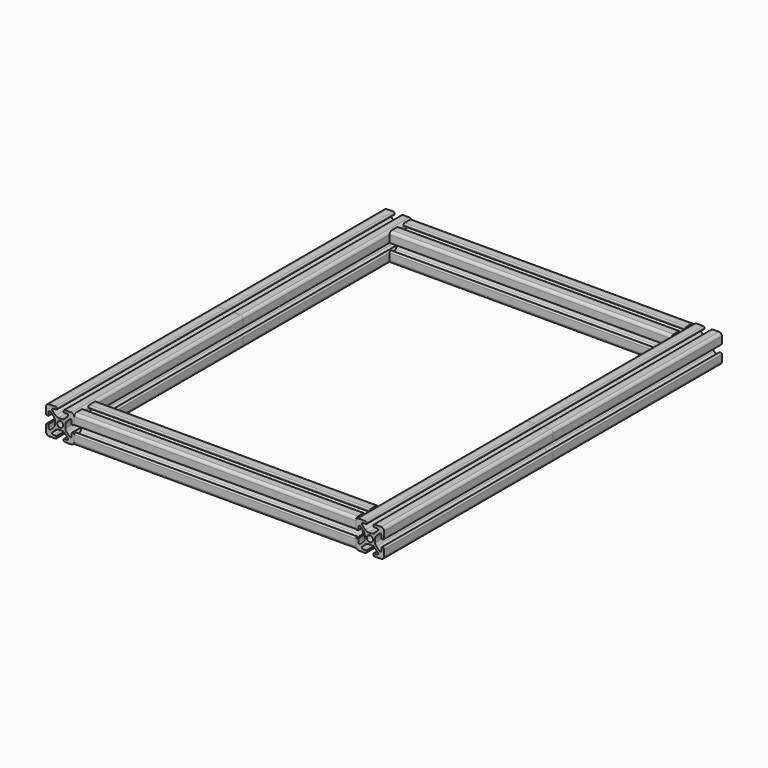
from build123d import *

# Parameters (mm, degrees)
F1_DEPTH = 150
F3_DEPTH = 100


# Not quite as in the source:
# - ends of sketch curves that miss each other by under 0.0002 mm in the source are joined


with BuildPart() as f1:
    # F0 (on Front) → F1 (new body, symmetric)
    with BuildSketch(Plane.XZ):
        with BuildLine():
            ThreePointArc((-112.15, 0), (-111.5202795796, 1.5202795796), (-110, 2.15))
            Line((-110, 2.15), (-110, 3.65))
            Line((-110, 3.65), (-111.134567, 3.65))
            ThreePointArc((-111.134567, 3.65), (-112.2826172971, 3.8783614025), (-113.2558873436, 4.5286796564))
            Line((-113.2558873436, 4.5286796564), (-115.506192, 6.778984))
            ThreePointArc((-115.506192, 6.778984), (-115.6866364094, 7.6861382813), (-114.917588, 8.2))
            Line((-114.917588, 8.2), (-112.8, 8.200001))
            ThreePointArc((-112.8, 8.200001), (-112.5878679656, 8.2878679656), (-112.5, 8.5))
            Line((-112.5, 8.5), (-112.5, 9.200001))
            ThreePointArc((-112.5, 9.200001), (-112.7343145751, 9.7656854249), (-113.3, 10))
            Line((-113.3, 10), (-118, 10))
            ThreePointArc((-118, 10), (-119.4142135624, 9.4142135624), (-120, 8))
            Line((-120, 8), (-120, 3.3))
            ThreePointArc((-120, 3.3), (-119.7656854249, 2.7343145751), (-119.2, 2.5))
            Line((-119.2, 2.5), (-118.5, 2.5))
            ThreePointArc((-118.5, 2.5), (-118.2878679656, 2.5878679656), (-118.2, 2.8))
            Line((-118.2, 2.8), (-118.2, 4.917588))
            ThreePointArc((-118.2, 4.917588), (-117.6861382813, 5.6866364094), (-116.7789838301, 5.5061921699))
            Line((-116.7789838301, 5.5061921699), (-114.52868, 3.255887))
            ThreePointArc((-114.52868, 3.255887), (-113.8783614025, 2.2826172971), (-113.65, 1.134567))
            Line((-113.65, 1.134567), (-113.65, 0))
            Line((-113.65, 0), (-112.15, 0))
        make_face()
        with BuildLine():
            Line((-107.85, 0), (-106.35, 0))
            Line((-106.35, 0), (-106.35, 1.134567))
            ThreePointArc((-106.35, 1.134567), (-106.1216385975, 2.2826172971), (-105.4713203436, 3.2558873436))
            Line((-105.4713203436, 3.2558873436), (-103.221016, 5.506192))
            ThreePointArc((-103.221016, 5.506192), (-102.3138617187, 5.6866364094), (-101.8, 4.917588))
            Line((-101.8, 4.917588), (-101.799999, 2.8))
            ThreePointArc((-101.799999, 2.8), (-101.7121320344, 2.5878679656), (-101.5, 2.5))
            Line((-101.5, 2.5), (-100.799999, 2.5))
            ThreePointArc((-100.799999, 2.5), (-100.2343145751, 2.7343145751), (-100, 3.3))
            Line((-100, 3.3), (-100, 8))
            ThreePointArc((-100, 8), (-100.5857864376, 9.4142135624), (-102, 10))
            Line((-102, 10), (-106.7, 10))
            ThreePointArc((-106.7, 10), (-107.2656854249, 9.7656854249), (-107.5, 9.2))
            Line((-107.5, 9.2), (-107.5, 8.5))
            ThreePointArc((-107.5, 8.5), (-107.4121320344, 8.2878679656), (-107.2, 8.2))
            Line((-107.2, 8.2), (-105.082412, 8.200001))
            ThreePointArc((-105.082412, 8.200001), (-104.3133635906, 7.6861382813), (-104.4938078301, 6.7789838301))
            Line((-104.4938078301, 6.7789838301), (-106.744113, 4.52868))
            ThreePointArc((-106.744113, 4.52868), (-107.7173827029, 3.8783614025), (-108.865433, 3.65))
            Line((-108.865433, 3.65), (-110, 3.65))
            Line((-110, 3.65), (-110, 2.15))
            ThreePointArc((-110, 2.15), (-108.4797204204, 1.5202795796), (-107.85, 0))
        make_face()
        with BuildLine():
            Line((-110, -3.65), (-110, -2.15))
            ThreePointArc((-110, -2.15), (-111.5202795796, -1.5202795796), (-112.15, 0))
            Line((-112.15, 0), (-113.65, 0))
            Line((-113.65, 0), (-113.65, -1.134567))
            ThreePointArc((-113.65, -1.134567), (-113.8783614025, -2.2826172971), (-114.5286796564, -3.2558873436))
            Line((-114.5286796564, -3.2558873436), (-116.778985, -5.506192))
            ThreePointArc((-116.778985, -5.506192), (-117.6861382813, -5.6866364094), (-118.2, -4.917588))
            Line((-118.2, -4.917588), (-118.2, -2.8))
            ThreePointArc((-118.2, -2.8), (-118.2878679656, -2.5878679656), (-118.5, -2.5))
            Line((-118.5, -2.5), (-119.2, -2.5))
            ThreePointArc((-119.2, -2.5), (-119.7656854249, -2.7343145751), (-120, -3.3))
            Line((-120, -3.3), (-120, -8))
            ThreePointArc((-120, -8), (-119.4142135624, -9.4142135624), (-118, -10))
            Line((-118, -10), (-113.3, -10))
            ThreePointArc((-113.3, -10), (-112.7343145751, -9.7656854249), (-112.5, -9.2))
            Line((-112.5, -9.2), (-112.5, -8.5))
            ThreePointArc((-112.5, -8.5), (-112.5878679656, -8.2878679656), (-112.8, -8.2))
            Line((-112.8, -8.2), (-114.917588, -8.2))
            ThreePointArc((-114.917588, -8.2), (-115.6866364094, -7.6861382813), (-115.5061921699, -6.7789838301))
            Line((-115.5061921699, -6.7789838301), (-113.255888, -4.52868))
            ThreePointArc((-113.255888, -4.52868), (-112.2826172971, -3.8783614025), (-111.134567, -3.65))
            Line((-111.134567, -3.65), (-110, -3.65))
        make_face()
        with BuildLine():
            ThreePointArc((-101.8, -4.917588), (-102.3138617187, -5.6866364094), (-103.2210161699, -5.5061921699))
            Line((-103.2210161699, -5.5061921699), (-105.47132, -3.255888))
            ThreePointArc((-105.47132, -3.255888), (-106.1216385975, -2.2826172971), (-106.35, -1.134567))
            Line((-106.35, -1.134567), (-106.35, 0))
            Line((-106.35, 0), (-107.85, 0))
            ThreePointArc((-107.85, 0), (-108.4797204204, -1.5202795796), (-110, -2.15))
            Line((-110, -2.15), (-110, -3.65))
            Line((-110, -3.65), (-108.865433, -3.65))
            ThreePointArc((-108.865433, -3.65), (-107.7173827029, -3.8783614025), (-106.7441126564, -4.5286796564))
            Line((-106.7441126564, -4.5286796564), (-104.493808, -6.778985))
            ThreePointArc((-104.493808, -6.778985), (-104.3133635906, -7.6861382813), (-105.082412, -8.2))
            Line((-105.082412, -8.2), (-107.2, -8.2))
            ThreePointArc((-107.2, -8.2), (-107.4121320344, -8.2878679656), (-107.5, -8.5))
            Line((-107.5, -8.5), (-107.5, -9.2))
            ThreePointArc((-107.5, -9.2), (-107.2656854249, -9.7656854249), (-106.7, -10))
            Line((-106.7, -10), (-102, -10))
            ThreePointArc((-102, -10), (-100.5857864376, -9.4142135624), (-100, -8))
            Line((-100, -8), (-100, -3.3))
            ThreePointArc((-100, -3.3), (-100.2343145751, -2.7343145751), (-100.8, -2.5))
            Line((-100.8, -2.5), (-101.5, -2.5))
            ThreePointArc((-101.5, -2.5), (-101.7121320344, -2.5878679656), (-101.8, -2.8))
            Line((-101.8, -2.8), (-101.8, -4.917588))
        make_face()
    extrude(amount=F1_DEPTH, both=True)


with BuildPart() as f1b:
    # F0 (on Front) → F1, piece 2 (new body, symmetric)
    with BuildSketch(Plane.XZ):
        with BuildLine():
            ThreePointArc((107.85, 0), (108.4797204204, 1.5202795796), (110, 2.15))
            Line((110, 2.15), (110, 3.65))
            Line((110, 3.65), (108.865433, 3.65))
            ThreePointArc((108.865433, 3.65), (107.7173827029, 3.8783614025), (106.7441126564, 4.5286796564))
            Line((106.7441126564, 4.5286796564), (104.493808, 6.778984))
            ThreePointArc((104.493808, 6.778984), (104.3133635906, 7.6861382813), (105.082412, 8.2))
            Line((105.082412, 8.2), (107.2, 8.200001))
            ThreePointArc((107.2, 8.200001), (107.4121320344, 8.2878679656), (107.5, 8.5))
            Line((107.5, 8.5), (107.5, 9.200001))
            ThreePointArc((107.5, 9.200001), (107.2656854249, 9.7656854249), (106.7, 10))
            Line((106.7, 10), (102, 10))
            ThreePointArc((102, 10), (100.5857864376, 9.4142135624), (100, 8))
            Line((100, 8), (100, 3.3))
            ThreePointArc((100, 3.3), (100.2343145751, 2.7343145751), (100.8, 2.5))
            Line((100.8, 2.5), (101.5, 2.5))
            ThreePointArc((101.5, 2.5), (101.7121320344, 2.5878679656), (101.8, 2.8))
            Line((101.8, 2.8), (101.8, 4.917588))
            ThreePointArc((101.8, 4.917588), (102.3138617187, 5.6866364094), (103.2210161699, 5.5061921699))
            Line((103.2210161699, 5.5061921699), (105.47132, 3.255887))
            ThreePointArc((105.47132, 3.255887), (106.1216385975, 2.2826172971), (106.35, 1.134567))
            Line((106.35, 1.134567), (106.35, 0))
            Line((106.35, 0), (107.85, 0))
        make_face()
        with BuildLine():
            Line((112.15, 0), (113.65, 0))
            Line((113.65, 0), (113.65, 1.134567))
            ThreePointArc((113.65, 1.134567), (113.8783614025, 2.2826172971), (114.5286796564, 3.2558873436))
            Line((114.5286796564, 3.2558873436), (116.778984, 5.506192))
            ThreePointArc((116.778984, 5.506192), (117.6861382813, 5.6866364094), (118.2, 4.917588))
            Line((118.2, 4.917588), (118.200001, 2.8))
            ThreePointArc((118.200001, 2.8), (118.2878679656, 2.5878679656), (118.5, 2.5))
            Line((118.5, 2.5), (119.200001, 2.5))
            ThreePointArc((119.200001, 2.5), (119.7656854249, 2.7343145751), (120, 3.3))
            Line((120, 3.3), (120, 8))
            ThreePointArc((120, 8), (119.4142135624, 9.4142135624), (118, 10))
            Line((118, 10), (113.3, 10))
            ThreePointArc((113.3, 10), (112.7343145751, 9.7656854249), (112.5, 9.2))
            Line((112.5, 9.2), (112.5, 8.5))
            ThreePointArc((112.5, 8.5), (112.5878679656, 8.2878679656), (112.8, 8.2))
            Line((112.8, 8.2), (114.917588, 8.200001))
            ThreePointArc((114.917588, 8.200001), (115.6866364094, 7.6861382813), (115.5061921699, 6.7789838301))
            Line((115.5061921699, 6.7789838301), (113.255887, 4.52868))
            ThreePointArc((113.255887, 4.52868), (112.2826172971, 3.8783614025), (111.134567, 3.65))
            Line((111.134567, 3.65), (110, 3.65))
            Line((110, 3.65), (110, 2.15))
            ThreePointArc((110, 2.15), (111.5202795796, 1.5202795796), (112.15, 0))
        make_face()
        with BuildLine():
            ThreePointArc((118.2, -4.917588), (117.6861382813, -5.6866364094), (116.7789838301, -5.5061921699))
            Line((116.7789838301, -5.5061921699), (114.52868, -3.255888))
            ThreePointArc((114.52868, -3.255888), (113.8783614025, -2.2826172971), (113.65, -1.134567))
            Line((113.65, -1.134567), (113.65, 0))
            Line((113.65, 0), (112.15, 0))
            ThreePointArc((112.15, 0), (111.5202795796, -1.5202795796), (110, -2.15))
            Line((110, -2.15), (110, -3.65))
            Line((110, -3.65), (111.134567, -3.65))
            ThreePointArc((111.134567, -3.65), (112.2826172971, -3.8783614025), (113.2558873436, -4.5286796564))
            Line((113.2558873436, -4.5286796564), (115.506192, -6.778985))
            ThreePointArc((115.506192, -6.778985), (115.6866364094, -7.6861382813), (114.917588, -8.2))
            Line((114.917588, -8.2), (112.8, -8.2))
            ThreePointArc((112.8, -8.2), (112.5878679656, -8.2878679656), (112.5, -8.5))
            Line((112.5, -8.5), (112.5, -9.2))
            ThreePointArc((112.5, -9.2), (112.7343145751, -9.7656854249), (113.3, -10))
            Line((113.3, -10), (118, -10))
            ThreePointArc((118, -10), (119.4142135624, -9.4142135624), (120, -8))
            Line((120, -8), (120, -3.3))
            ThreePointArc((120, -3.3), (119.7656854249, -2.7343145751), (119.2, -2.5))
            Line((119.2, -2.5), (118.5, -2.5))
            ThreePointArc((118.5, -2.5), (118.2878679656, -2.5878679656), (118.2, -2.8))
            Line((118.2, -2.8), (118.2, -4.917588))
        make_face()
        with BuildLine():
            Line((110, -3.65), (110, -2.15))
            ThreePointArc((110, -2.15), (108.4797204204, -1.5202795796), (107.85, 0))
            Line((107.85, 0), (106.35, 0))
            Line((106.35, 0), (106.35, -1.134567))
            ThreePointArc((106.35, -1.134567), (106.1216385975, -2.2826172971), (105.4713203436, -3.2558873436))
            Line((105.4713203436, -3.2558873436), (103.221015, -5.506192))
            ThreePointArc((103.221015, -5.506192), (102.3138617187, -5.6866364094), (101.8, -4.917588))
            Line((101.8, -4.917588), (101.8, -2.8))
            ThreePointArc((101.8, -2.8), (101.7121320344, -2.5878679656), (101.5, -2.5))
            Line((101.5, -2.5), (100.8, -2.5))
            ThreePointArc((100.8, -2.5), (100.2343145751, -2.7343145751), (100, -3.3))
            Line((100, -3.3), (100, -8))
            ThreePointArc((100, -8), (100.5857864376, -9.4142135624), (102, -10))
            Line((102, -10), (106.7, -10))
            ThreePointArc((106.7, -10), (107.2656854249, -9.7656854249), (107.5, -9.2))
            Line((107.5, -9.2), (107.5, -8.5))
            ThreePointArc((107.5, -8.5), (107.4121320344, -8.2878679656), (107.2, -8.2))
            Line((107.2, -8.2), (105.082412, -8.2))
            ThreePointArc((105.082412, -8.2), (104.3133635906, -7.6861382813), (104.4938078301, -6.7789838301))
            Line((104.4938078301, -6.7789838301), (106.744112, -4.52868))
            ThreePointArc((106.744112, -4.52868), (107.7173827029, -3.8783614025), (108.865433, -3.65))
            Line((108.865433, -3.65), (110, -3.65))
        make_face()
    extrude(amount=F1_DEPTH, both=True)


with BuildPart() as f3:
    # F2 (on Right) → F3 (new body, symmetric)
    with BuildSketch(Plane.YZ):
        with BuildLine():
            ThreePointArc((-131.8, -4.917588), (-132.3138617187, -5.6866364094), (-133.2210161699, -5.5061921699))
            Line((-133.2210161699, -5.5061921699), (-135.47132, -3.255888))
            ThreePointArc((-135.47132, -3.255888), (-136.1216385975, -2.2826172971), (-136.35, -1.134567))
            Line((-136.35, -1.134567), (-136.35, 0))
            Line((-136.35, 0), (-137.85, 0))
            ThreePointArc((-137.85, 0), (-138.4797204204, -1.5202795796), (-140, -2.15))
            Line((-140, -2.15), (-140, -3.65))
            Line((-140, -3.65), (-138.865433, -3.65))
            ThreePointArc((-138.865433, -3.65), (-137.7173827029, -3.8783614025), (-136.7441126564, -4.5286796564))
            Line((-136.7441126564, -4.5286796564), (-134.493808, -6.778985))
            ThreePointArc((-134.493808, -6.778985), (-134.3133635906, -7.6861382813), (-135.082412, -8.2))
            Line((-135.082412, -8.2), (-137.2, -8.2))
            ThreePointArc((-137.2, -8.2), (-137.4121320344, -8.2878679656), (-137.5, -8.5))
            Line((-137.5, -8.5), (-137.5, -9.2))
            ThreePointArc((-137.5, -9.2), (-137.2656854249, -9.7656854249), (-136.7, -10))
            Line((-136.7, -10), (-132, -10))
            ThreePointArc((-132, -10), (-130.5857864376, -9.4142135624), (-130, -8))
            Line((-130, -8), (-130, -3.3))
            ThreePointArc((-130, -3.3), (-130.2343145751, -2.7343145751), (-130.8, -2.5))
            Line((-130.8, -2.5), (-131.5, -2.5))
            ThreePointArc((-131.5, -2.5), (-131.7121320344, -2.5878679656), (-131.8, -2.8))
            Line((-131.8, -2.8), (-131.8, -4.917588))
        make_face()
        with BuildLine():
            Line((-137.85, 0), (-136.35, 0))
            Line((-136.35, 0), (-136.35, 1.134567))
            ThreePointArc((-136.35, 1.134567), (-136.1216385975, 2.2826172971), (-135.4713203436, 3.2558873436))
            Line((-135.4713203436, 3.2558873436), (-133.221016, 5.506192))
            ThreePointArc((-133.221016, 5.506192), (-132.3138617187, 5.6866364094), (-131.8, 4.917588))
            Line((-131.8, 4.917588), (-131.799999, 2.8))
            ThreePointArc((-131.799999, 2.8), (-131.7121320344, 2.5878679656), (-131.5, 2.5))
            Line((-131.5, 2.5), (-130.799999, 2.5))
            ThreePointArc((-130.799999, 2.5), (-130.2343145751, 2.7343145751), (-130, 3.3))
            Line((-130, 3.3), (-130, 8))
            ThreePointArc((-130, 8), (-130.5857864376, 9.4142135624), (-132, 10))
            Line((-132, 10), (-136.7, 10))
            ThreePointArc((-136.7, 10), (-137.2656854249, 9.7656854249), (-137.5, 9.2))
            Line((-137.5, 9.2), (-137.5, 8.5))
            ThreePointArc((-137.5, 8.5), (-137.4121320344, 8.2878679656), (-137.2, 8.2))
            Line((-137.2, 8.2), (-135.082412, 8.200001))
            ThreePointArc((-135.082412, 8.200001), (-134.3133635906, 7.6861382813), (-134.4938078301, 6.7789838301))
            Line((-134.4938078301, 6.7789838301), (-136.744113, 4.52868))
            ThreePointArc((-136.744113, 4.52868), (-137.7173827029, 3.8783614025), (-138.865433, 3.65))
            Line((-138.865433, 3.65), (-140, 3.65))
            Line((-140, 3.65), (-140, 2.15))
            ThreePointArc((-140, 2.15), (-138.4797204204, 1.5202795796), (-137.85, 0))
        make_face()
        with BuildLine():
            ThreePointArc((-142.15, 0), (-141.5202795796, 1.5202795796), (-140, 2.15))
            Line((-140, 2.15), (-140, 3.65))
            Line((-140, 3.65), (-141.134567, 3.65))
            ThreePointArc((-141.134567, 3.65), (-142.2826172971, 3.8783614025), (-143.2558873436, 4.5286796564))
            Line((-143.2558873436, 4.5286796564), (-145.506192, 6.778984))
            ThreePointArc((-145.506192, 6.778984), (-145.6866364094, 7.6861382813), (-144.917588, 8.2))
            Line((-144.917588, 8.2), (-142.8, 8.200001))
            ThreePointArc((-142.8, 8.200001), (-142.5878679656, 8.2878679656), (-142.5, 8.5))
            Line((-142.5, 8.5), (-142.5, 9.200001))
            ThreePointArc((-142.5, 9.200001), (-142.7343145751, 9.7656854249), (-143.3, 10))
            Line((-143.3, 10), (-148, 10))
            ThreePointArc((-148, 10), (-149.4142135624, 9.4142135624), (-150, 8))
            Line((-150, 8), (-150, 3.3))
            ThreePointArc((-150, 3.3), (-149.7656854249, 2.7343145751), (-149.2, 2.5))
            Line((-149.2, 2.5), (-148.5, 2.5))
            ThreePointArc((-148.5, 2.5), (-148.2878679656, 2.5878679656), (-148.2, 2.8))
            Line((-148.2, 2.8), (-148.2, 4.917588))
            ThreePointArc((-148.2, 4.917588), (-147.6861382813, 5.6866364094), (-146.7789838301, 5.5061921699))
            Line((-146.7789838301, 5.5061921699), (-144.52868, 3.255887))
            ThreePointArc((-144.52868, 3.255887), (-143.8783614025, 2.2826172971), (-143.65, 1.134567))
            Line((-143.65, 1.134567), (-143.65, 0))
            Line((-143.65, 0), (-142.15, 0))
        make_face()
        with BuildLine():
            Line((-140, -3.65), (-140, -2.15))
            ThreePointArc((-140, -2.15), (-141.5202795796, -1.5202795796), (-142.15, 0))
            Line((-142.15, 0), (-143.65, 0))
            Line((-143.65, 0), (-143.65, -1.134567))
            ThreePointArc((-143.65, -1.134567), (-143.8783614025, -2.2826172971), (-144.5286796564, -3.2558873436))
            Line((-144.5286796564, -3.2558873436), (-146.778985, -5.506192))
            ThreePointArc((-146.778985, -5.506192), (-147.6861382813, -5.6866364094), (-148.2, -4.917588))
            Line((-148.2, -4.917588), (-148.2, -2.8))
            ThreePointArc((-148.2, -2.8), (-148.2878679656, -2.5878679656), (-148.5, -2.5))
            Line((-148.5, -2.5), (-149.2, -2.5))
            ThreePointArc((-149.2, -2.5), (-149.7656854249, -2.7343145751), (-150, -3.3))
            Line((-150, -3.3), (-150, -8))
            ThreePointArc((-150, -8), (-149.4142135624, -9.4142135624), (-148, -10))
            Line((-148, -10), (-143.3, -10))
            ThreePointArc((-143.3, -10), (-142.7343145751, -9.7656854249), (-142.5, -9.2))
            Line((-142.5, -9.2), (-142.5, -8.5))
            ThreePointArc((-142.5, -8.5), (-142.5878679656, -8.2878679656), (-142.8, -8.2))
            Line((-142.8, -8.2), (-144.917588, -8.2))
            ThreePointArc((-144.917588, -8.2), (-145.6866364094, -7.6861382813), (-145.5061921699, -6.7789838301))
            Line((-145.5061921699, -6.7789838301), (-143.255888, -4.52868))
            ThreePointArc((-143.255888, -4.52868), (-142.2826172971, -3.8783614025), (-141.134567, -3.65))
            Line((-141.134567, -3.65), (-140, -3.65))
        make_face()
    extrude(amount=F3_DEPTH, both=True)


with BuildPart() as f3b:
    # F2 (on Right) → F3, piece 2 (new body, symmetric)
    with BuildSketch(Plane.YZ):
        with BuildLine():
            ThreePointArc((148.2, -4.917588), (147.6861382813, -5.6866364094), (146.7789838301, -5.5061921699))
            Line((146.7789838301, -5.5061921699), (144.52868, -3.255888))
            ThreePointArc((144.52868, -3.255888), (143.8783614025, -2.2826172971), (143.65, -1.134567))
            Line((143.65, -1.134567), (143.65, 0))
            Line((143.65, 0), (142.15, 0))
            ThreePointArc((142.15, 0), (141.5202795796, -1.5202795796), (140, -2.15))
            Line((140, -2.15), (140, -3.65))
            Line((140, -3.65), (141.134567, -3.65))
            ThreePointArc((141.134567, -3.65), (142.2826172971, -3.8783614025), (143.2558873436, -4.5286796564))
            Line((143.2558873436, -4.5286796564), (145.506192, -6.778985))
            ThreePointArc((145.506192, -6.778985), (145.6866364094, -7.6861382813), (144.917588, -8.2))
            Line((144.917588, -8.2), (142.8, -8.2))
            ThreePointArc((142.8, -8.2), (142.5878679656, -8.2878679656), (142.5, -8.5))
            Line((142.5, -8.5), (142.5, -9.2))
            ThreePointArc((142.5, -9.2), (142.7343145751, -9.7656854249), (143.3, -10))
            Line((143.3, -10), (148, -10))
            ThreePointArc((148, -10), (149.4142135624, -9.4142135624), (150, -8))
            Line((150, -8), (150, -3.3))
            ThreePointArc((150, -3.3), (149.7656854249, -2.7343145751), (149.2, -2.5))
            Line((149.2, -2.5), (148.5, -2.5))
            ThreePointArc((148.5, -2.5), (148.2878679656, -2.5878679656), (148.2, -2.8))
            Line((148.2, -2.8), (148.2, -4.917588))
        make_face()
        with BuildLine():
            Line((142.15, 0), (143.65, 0))
            Line((143.65, 0), (143.65, 1.134567))
            ThreePointArc((143.65, 1.134567), (143.8783614025, 2.2826172971), (144.5286796564, 3.2558873436))
            Line((144.5286796564, 3.2558873436), (146.778984, 5.506192))
            ThreePointArc((146.778984, 5.506192), (147.6861382813, 5.6866364094), (148.2, 4.917588))
            Line((148.2, 4.917588), (148.200001, 2.8))
            ThreePointArc((148.200001, 2.8), (148.2878679656, 2.5878679656), (148.5, 2.5))
            Line((148.5, 2.5), (149.200001, 2.5))
            ThreePointArc((149.200001, 2.5), (149.7656854249, 2.7343145751), (150, 3.3))
            Line((150, 3.3), (150, 8))
            ThreePointArc((150, 8), (149.4142135624, 9.4142135624), (148, 10))
            Line((148, 10), (143.3, 10))
            ThreePointArc((143.3, 10), (142.7343145751, 9.7656854249), (142.5, 9.2))
            Line((142.5, 9.2), (142.5, 8.5))
            ThreePointArc((142.5, 8.5), (142.5878679656, 8.2878679656), (142.8, 8.2))
            Line((142.8, 8.2), (144.917588, 8.200001))
            ThreePointArc((144.917588, 8.200001), (145.6866364094, 7.6861382813), (145.5061921699, 6.7789838301))
            Line((145.5061921699, 6.7789838301), (143.255887, 4.52868))
            ThreePointArc((143.255887, 4.52868), (142.2826172971, 3.8783614025), (141.134567, 3.65))
            Line((141.134567, 3.65), (140, 3.65))
            Line((140, 3.65), (140, 2.15))
            ThreePointArc((140, 2.15), (141.5202795796, 1.5202795796), (142.15, 0))
        make_face()
        with BuildLine():
            ThreePointArc((137.85, 0), (138.4797204204, 1.5202795796), (140, 2.15))
            Line((140, 2.15), (140, 3.65))
            Line((140, 3.65), (138.865433, 3.65))
            ThreePointArc((138.865433, 3.65), (137.7173827029, 3.8783614025), (136.7441126564, 4.5286796564))
            Line((136.7441126564, 4.5286796564), (134.493808, 6.778984))
            ThreePointArc((134.493808, 6.778984), (134.3133635906, 7.6861382813), (135.082412, 8.2))
            Line((135.082412, 8.2), (137.2, 8.200001))
            ThreePointArc((137.2, 8.200001), (137.4121320344, 8.2878679656), (137.5, 8.5))
            Line((137.5, 8.5), (137.5, 9.200001))
            ThreePointArc((137.5, 9.200001), (137.2656854249, 9.7656854249), (136.7, 10))
            Line((136.7, 10), (132, 10))
            ThreePointArc((132, 10), (130.5857864376, 9.4142135624), (130, 8))
            Line((130, 8), (130, 3.3))
            ThreePointArc((130, 3.3), (130.2343145751, 2.7343145751), (130.8, 2.5))
            Line((130.8, 2.5), (131.5, 2.5))
            ThreePointArc((131.5, 2.5), (131.7121320344, 2.5878679656), (131.8, 2.8))
            Line((131.8, 2.8), (131.8, 4.917588))
            ThreePointArc((131.8, 4.917588), (132.3138617187, 5.6866364094), (133.2210161699, 5.5061921699))
            Line((133.2210161699, 5.5061921699), (135.47132, 3.255887))
            ThreePointArc((135.47132, 3.255887), (136.1216385975, 2.2826172971), (136.35, 1.134567))
            Line((136.35, 1.134567), (136.35, 0))
            Line((136.35, 0), (137.85, 0))
        make_face()
        with BuildLine():
            Line((140, -3.65), (140, -2.15))
            ThreePointArc((140, -2.15), (138.4797204204, -1.5202795796), (137.85, 0))
            Line((137.85, 0), (136.35, 0))
            Line((136.35, 0), (136.35, -1.134567))
            ThreePointArc((136.35, -1.134567), (136.1216385975, -2.2826172971), (135.4713203436, -3.2558873436))
            Line((135.4713203436, -3.2558873436), (133.221015, -5.506192))
            ThreePointArc((133.221015, -5.506192), (132.3138617187, -5.6866364094), (131.8, -4.917588))
            Line((131.8, -4.917588), (131.8, -2.8))
            ThreePointArc((131.8, -2.8), (131.7121320344, -2.5878679656), (131.5, -2.5))
            Line((131.5, -2.5), (130.8, -2.5))
            ThreePointArc((130.8, -2.5), (130.2343145751, -2.7343145751), (130, -3.3))
            Line((130, -3.3), (130, -8))
            ThreePointArc((130, -8), (130.5857864376, -9.4142135624), (132, -10))
            Line((132, -10), (136.7, -10))
            ThreePointArc((136.7, -10), (137.2656854249, -9.7656854249), (137.5, -9.2))
            Line((137.5, -9.2), (137.5, -8.5))
            ThreePointArc((137.5, -8.5), (137.4121320344, -8.2878679656), (137.2, -8.2))
            Line((137.2, -8.2), (135.082412, -8.2))
            ThreePointArc((135.082412, -8.2), (134.3133635906, -7.6861382813), (134.4938078301, -6.7789838301))
            Line((134.4938078301, -6.7789838301), (136.744112, -4.52868))
            ThreePointArc((136.744112, -4.52868), (137.7173827029, -3.8783614025), (138.865433, -3.65))
            Line((138.865433, -3.65), (140, -3.65))
        make_face()
    extrude(amount=F3_DEPTH, both=True)


solid = Compound([f1.part, f1b.part, f3.part, f3b.part])
